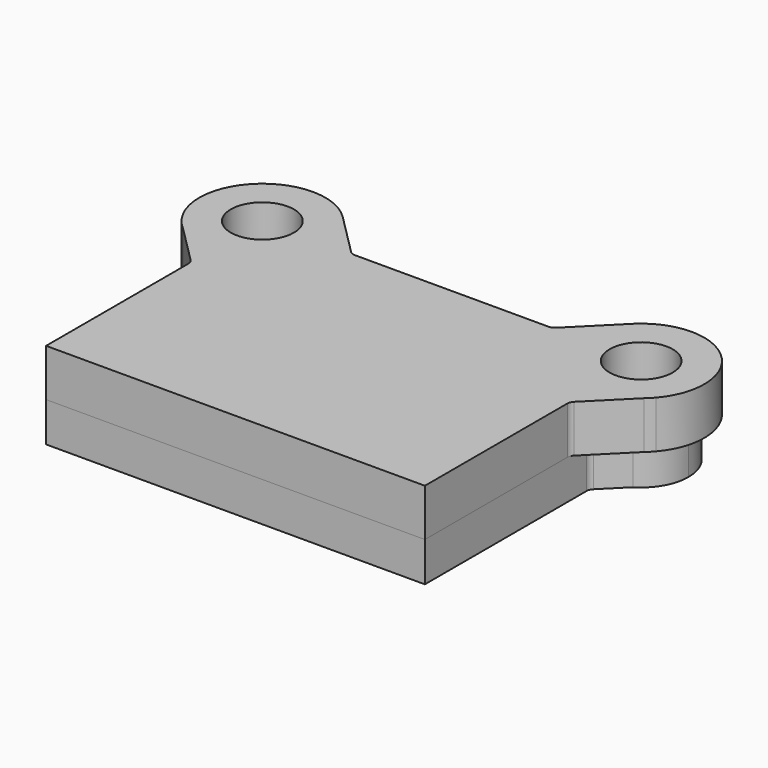
from build123d import *

# Parameters (mm, degrees)
F0_R     = 25.4
F1_DEPTH = 31.75
F4_R     = 25.4
F5_DEPTH = 38.1
F7_DEPTH = 25.4


with BuildPart() as f1:
    # F0 (on Top) → F1 (new body)
    with BuildSketch(Plane.XY):
        with BuildLine():
            Line((-152.4, 53.9033839703), (-152.4, -108.7667216295))
            Line((-152.4, -108.7667216295), (152.4, -108.7667216295))
            Line((152.4, -108.7667216295), (152.4, 53.9033839703))
            ThreePointArc((152.4, 53.9033839703), (152.8833649686, 56.3334237658), (154.2598719395, 58.3935120309))
            Line((154.2598719395, 58.3935120309), (171.9035763614, 76.0372164528))
            ThreePointArc((171.9035763614, 76.0372164528), (125.6457900901, 81.6406778321), (119.4044321158, 127.8167216295))
            Line((119.4044321158, 127.8167216295), (102.2143040553, 110.626593569))
            ThreePointArc((102.2143040553, 110.626593569), (100.1542157903, 109.2500865981), (97.7241759947, 108.7667216295))
            Line((97.7241759947, 108.7667216295), (-97.7241759947, 108.7667216295))
            ThreePointArc((-97.7241759947, 108.7667216295), (-100.1542157903, 109.2500865981), (-102.2143040553, 110.626593569))
            Line((-102.2143040553, 110.626593569), (-119.4044321158, 127.8167216295))
            ThreePointArc((-119.4044321158, 127.8167216295), (-115.5982260184, 118.6277272479), (-114.3, 108.7667216295))
            ThreePointArc((-114.3, 108.7667216295), (-125.4592316368, 81.8259532663), (-152.4, 70.6667216295))
            Line((-152.4, 70.6667216295), (-152.4, 53.9033839703))
        make_face()
        with BuildLine():
            ThreePointArc((-171.9035763614, 76.0372164528), (-162.5147380778, 72.0338742907), (-152.4, 70.6667216295))
            ThreePointArc((-152.4, 70.6667216295), (-125.4592316368, 81.8259532663), (-114.3, 108.7667216295))
            ThreePointArc((-114.3, 108.7667216295), (-115.5982260184, 118.6277272479), (-119.4044321158, 127.8167216295))
            ThreePointArc((-119.4044321158, 127.8167216295), (-179.1542099099, 135.8927654269), (-171.9035763614, 76.0372164528))
        make_face()
        with Locations((-152.4, 108.7667216295)):
            Circle(F0_R, mode=Mode.SUBTRACT)
        with BuildLine():
            ThreePointArc((119.4044321158, 127.8167216295), (125.6457900901, 81.6406778321), (171.9035763614, 76.0372164528))
            ThreePointArc((171.9035763614, 76.0372164528), (185.5262453303, 89.9448760687), (190.5, 108.7667216295))
            ThreePointArc((190.5, 108.7667216295), (162.2610056184, 145.5684956111), (119.4044321158, 127.8167216295))
        make_face()
        with Locations((152.4, 108.7667216295)):
            Circle(F0_R, mode=Mode.SUBTRACT)
        with BuildLine():
            ThreePointArc((-154.2598719395, 58.3935120309), (-152.8833649686, 56.3334237658), (-152.4, 53.9033839703))
            Line((-152.4, 53.9033839703), (-152.4, 70.6667216295))
            ThreePointArc((-152.4, 70.6667216295), (-162.5147380778, 72.0338742907), (-171.9035763614, 76.0372164528))
            Line((-171.9035763614, 76.0372164528), (-154.2598719395, 58.3935120309))
        make_face()
    extrude(amount=F1_DEPTH)


with BuildPart() as f2_1:
    # F2: copy of F1
    add(f1.part)


with BuildPart() as f5:
    # F4 (on face) → F5 (new body)
    with BuildSketch(Plane.XY.offset(31.75)):
        with BuildLine():
            Line((-152.4, -108.7667216295), (152.4, -108.7667216295))
            Line((152.4, -108.7667216295), (152.4, 34.487204177))
            ThreePointArc((152.4, 34.487204177), (152.8833649686, 36.9172439725), (154.2598719395, 38.9773322375))
            Line((154.2598719395, 38.9773322375), (185.5948326386, 70.3122929367))
            Line((185.5948326386, 70.3122929367), (190.8544286929, 75.5718889909))
            ThreePointArc((190.8544286929, 75.5718889909), (187.3817017696, 145.6031240231), (117.2645696221, 145.4565231029))
            Line((117.2645696221, 145.4565231029), (115.7101985266, 143.9021520075))
            Line((115.7101985266, 143.9021520075), (82.4346400881, 110.626593569))
            ThreePointArc((82.4346400881, 110.626593569), (80.3745518231, 109.2500865981), (77.9445120276, 108.7667216295))
            Line((77.9445120276, 108.7667216295), (-77.9445120276, 108.7667216295))
            ThreePointArc((-77.9445120276, 108.7667216295), (-80.3745518231, 109.2500865981), (-82.4346400881, 110.626593569))
            Line((-82.4346400881, 110.626593569), (-115.7101985266, 143.9021520075))
            Line((-115.7101985266, 143.9021520075), (-117.2645696221, 145.4565231029))
            ThreePointArc((-117.2645696221, 145.4565231029), (-187.3817017696, 145.6031240231), (-190.8544286929, 75.5718889909))
            Line((-190.8544286929, 75.5718889909), (-185.5948326386, 70.3122929367))
            Line((-185.5948326386, 70.3122929367), (-154.2598719395, 38.9773322375))
            ThreePointArc((-154.2598719395, 38.9773322375), (-152.8833649686, 36.9172439725), (-152.4, 34.487204177))
            Line((-152.4, 34.487204177), (-152.4, -108.7667216295))
        make_face()
        with Locations((-152.4, 108.7667216295)):
            Circle(F4_R, mode=Mode.SUBTRACT)
        with Locations((152.4, 108.7667216295)):
            Circle(F4_R, mode=Mode.SUBTRACT)
        with BuildLine():
            Line((190.8544286929, 75.5718889909), (185.5948326386, 70.3122929367))
            ThreePointArc((185.5948326386, 70.3122929367), (188.3210244843, 72.8456971453), (190.8544286929, 75.5718889909))
        make_face()
        with BuildLine():
            ThreePointArc((-190.8544286929, 75.5718889909), (-188.3210244843, 72.8456971453), (-185.5948326386, 70.3122929367))
            Line((-185.5948326386, 70.3122929367), (-190.8544286929, 75.5718889909))
        make_face()
        with BuildLine():
            Line((115.7101985266, 143.9021520075), (117.2645696221, 145.4565231029))
            ThreePointArc((117.2645696221, 145.4565231029), (116.4789755157, 144.6877461138), (115.7101985266, 143.9021520075))
        make_face()
        with BuildLine():
            ThreePointArc((-115.7101985266, 143.9021520075), (-116.4789755157, 144.6877461138), (-117.2645696221, 145.4565231029))
            Line((-117.2645696221, 145.4565231029), (-115.7101985266, 143.9021520075))
        make_face()
    extrude(amount=F5_DEPTH)


with BuildPart() as f1_1:
    add(f1.part)

    # F6 (on Top) → F7 (cut)
    with BuildSketch(Plane.XY):
        with BuildLine():
            ThreePointArc((-19.050831298, -48.2122973633), (-15.4048473129, -46.7020813484), (-13.894631298, -43.0560973633))
            Line((-13.894631298, -43.0560973633), (-19.050831298, -43.0560973633))
            Line((-19.050831298, -43.0560973633), (-19.050831298, -48.2122973633))
        make_face()
        with BuildLine():
            ThreePointArc((-24.207031298, -43.0560973633), (-22.6968152832, -46.7020813484), (-19.050831298, -48.2122973633))
            Line((-19.050831298, -48.2122973633), (-19.050831298, -43.0560973633))
            Line((-19.050831298, -43.0560973633), (-24.207031298, -43.0560973633))
        make_face()
        with BuildLine():
            Line((-24.207031298, -43.0560973633), (-19.050831298, -43.0560973633))
            Line((-19.050831298, -43.0560973633), (-19.050831298, -37.8998973633))
            ThreePointArc((-19.050831298, -37.8998973633), (-22.6968152832, -39.4101133781), (-24.207031298, -43.0560973633))
        make_face()
        with BuildLine():
            Line((-19.050831298, -43.0560973633), (-13.894631298, -43.0560973633))
            ThreePointArc((-13.894631298, -43.0560973633), (-15.4048473129, -39.4101133781), (-19.050831298, -37.8998973633))
            Line((-19.050831298, -37.8998973633), (-19.050831298, -43.0560973633))
        make_face()
        with BuildLine():
            ThreePointArc((19.049168702, -47.8185973633), (22.4167647474, -46.4236934087), (23.811668702, -43.0560973633))
            Line((23.811668702, -43.0560973633), (19.049168702, -43.0560973633))
            Line((19.049168702, -43.0560973633), (19.049168702, -47.8185973633))
        make_face()
        with BuildLine():
            Line((19.049168702, -47.8185973633), (19.049168702, -43.0560973633))
            Line((19.049168702, -43.0560973633), (14.286668702, -43.0560973633))
            ThreePointArc((14.286668702, -43.0560973633), (15.6815726566, -46.4236934087), (19.049168702, -47.8185973633))
        make_face()
        with BuildLine():
            Line((14.286668702, -43.0560973633), (19.049168702, -43.0560973633))
            Line((19.049168702, -43.0560973633), (19.049168702, -38.2935973633))
            ThreePointArc((19.049168702, -38.2935973633), (15.6815726566, -39.6885013179), (14.286668702, -43.0560973633))
        make_face()
        with BuildLine():
            Line((19.049168702, -43.0560973633), (23.811668702, -43.0560973633))
            ThreePointArc((23.811668702, -43.0560973633), (22.4167647474, -39.6885013179), (19.049168702, -38.2935973633))
            Line((19.049168702, -38.2935973633), (19.049168702, -43.0560973633))
        make_face()
        with BuildLine():
            Line((19.049168702, 40.6877026367), (19.049168702, 45.8439026367))
            Line((19.049168702, 45.8439026367), (13.892968702, 45.8439026367))
            ThreePointArc((13.892968702, 45.8439026367), (15.4031847168, 42.1979186516), (19.049168702, 40.6877026367))
        make_face()
        with BuildLine():
            Line((19.049168702, 45.8439026367), (19.049168702, 51.0001026367))
            ThreePointArc((19.049168702, 51.0001026367), (15.4031847168, 49.4898866219), (13.892968702, 45.8439026367))
            Line((13.892968702, 45.8439026367), (19.049168702, 45.8439026367))
        make_face()
        with BuildLine():
            Line((19.049168702, 45.8439026367), (24.205368702, 45.8439026367))
            ThreePointArc((24.205368702, 45.8439026367), (22.6951526871, 49.4898866219), (19.049168702, 51.0001026367))
            Line((19.049168702, 51.0001026367), (19.049168702, 45.8439026367))
        make_face()
        with BuildLine():
            ThreePointArc((19.049168702, 40.6877026367), (22.6951526871, 42.1979186516), (24.205368702, 45.8439026367))
            Line((24.205368702, 45.8439026367), (19.049168702, 45.8439026367))
            Line((19.049168702, 45.8439026367), (19.049168702, 40.6877026367))
        make_face()
        with BuildLine():
            Line((-14.288331298, 45.8439026367), (-19.050831298, 45.8439026367))
            Line((-19.050831298, 45.8439026367), (-19.050831298, 41.0814026367))
            ThreePointArc((-19.050831298, 41.0814026367), (-15.6832352526, 42.4763065913), (-14.288331298, 45.8439026367))
        make_face()
        with BuildLine():
            ThreePointArc((-14.288331298, 45.8439026367), (-15.6832352526, 49.2114986821), (-19.050831298, 50.6064026367))
            Line((-19.050831298, 50.6064026367), (-19.050831298, 45.8439026367))
            Line((-19.050831298, 45.8439026367), (-14.288331298, 45.8439026367))
        make_face()
        with BuildLine():
            Line((-19.050831298, 45.8439026367), (-19.050831298, 50.6064026367))
            ThreePointArc((-19.050831298, 50.6064026367), (-22.4184273434, 49.2114986821), (-23.813331298, 45.8439026367))
            Line((-23.813331298, 45.8439026367), (-19.050831298, 45.8439026367))
        make_face()
        with BuildLine():
            Line((-19.050831298, 41.0814026367), (-19.050831298, 45.8439026367))
            Line((-19.050831298, 45.8439026367), (-23.813331298, 45.8439026367))
            ThreePointArc((-23.813331298, 45.8439026367), (-22.4184273434, 42.4763065913), (-19.050831298, 41.0814026367))
        make_face()
    extrude(amount=F7_DEPTH, mode=Mode.SUBTRACT)


solid = Compound([f5.part, f1_1.part])
